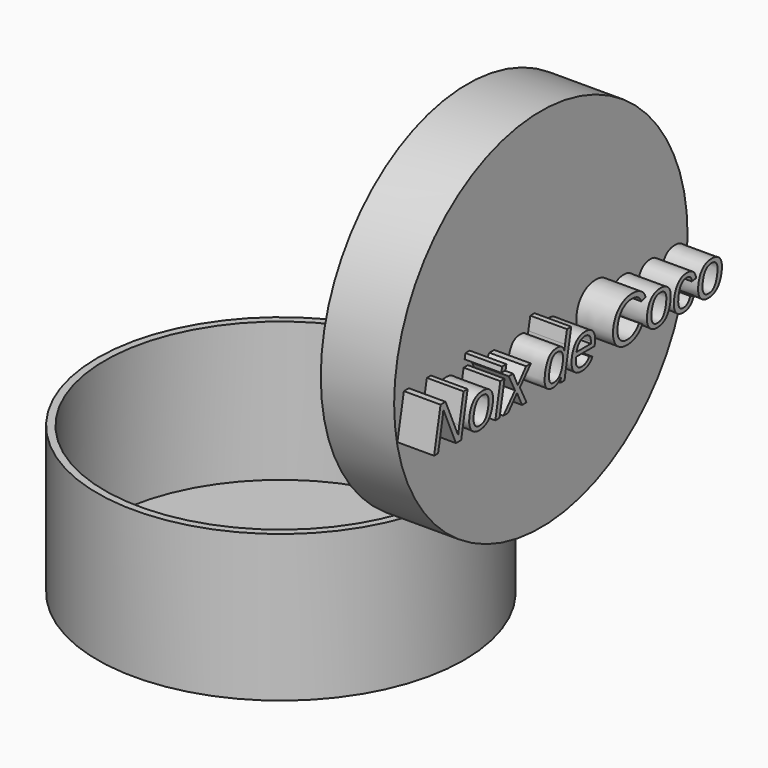
from build123d import *

# Parameters (mm, degrees)
F0_R         = 63.5
F1_DEPTH     = 50.8
F2_T         = -2.54
F3_R         = 63.5
F4_DEPTH     = 25.4
F5_T         = -2.54
F6_DEPTH     = 2.54
F7_TEXT_SIZE = 20.9743674431
F8_DEPTH     = 12.7


# Not quite as in the source:
# - Text() gives the source's letters only with a copy of the font that has no kerning and outlines rounded to 1/6400 em; it was checked with that copy


with BuildPart() as f1:
    # F0 (on Top) → F1 (new body)
    with BuildSketch(Plane.XY):
        with Locations((-63.9825984836, -98.7152904272)):
            Circle(F0_R)
    extrude(amount=F1_DEPTH)

    # F2
    f2_openings = [f1.faces().sort_by_distance(p)[0] for p in [
        (-63.982598, -98.71529, 50.8),
    ]]
    offset(amount=F2_T, openings=f2_openings)


with BuildPart() as f4:
    # F3 (on Right) → F4 (new body)
    with BuildSketch(Plane.YZ):
        with Locations((-97.9199334979, 111.9369417429)):
            Circle(F3_R)
    extrude(amount=F4_DEPTH)

    # F5
    f5_openings = [f4.faces().sort_by_distance(p)[0] for p in [
        (0, -97.919933, 111.936942),
    ]]
    offset(amount=F5_T, openings=f5_openings)

    # F6 (add): a face of the model
    f6_faces = [f4.faces().sort_by_distance(p)[0] for p in [
        (22.86, -97.9199334979, 111.9369417429),
    ]]
    extrude(f6_faces, amount=F6_DEPTH)

    # F7 (on face) → F8 (join)
    with BuildSketch(Plane.YZ.offset(25.4)):
        with Locations((-160.6457829475, 99.7215434909)):
            Text('Noix de Coco', F7_TEXT_SIZE, font='Arimo', font_style=FontStyle.ITALIC, text_align=(TextAlign.LEFT, TextAlign.BOTTOM))
    extrude(amount=F8_DEPTH)


solid = Compound([f1.part, f4.part])
